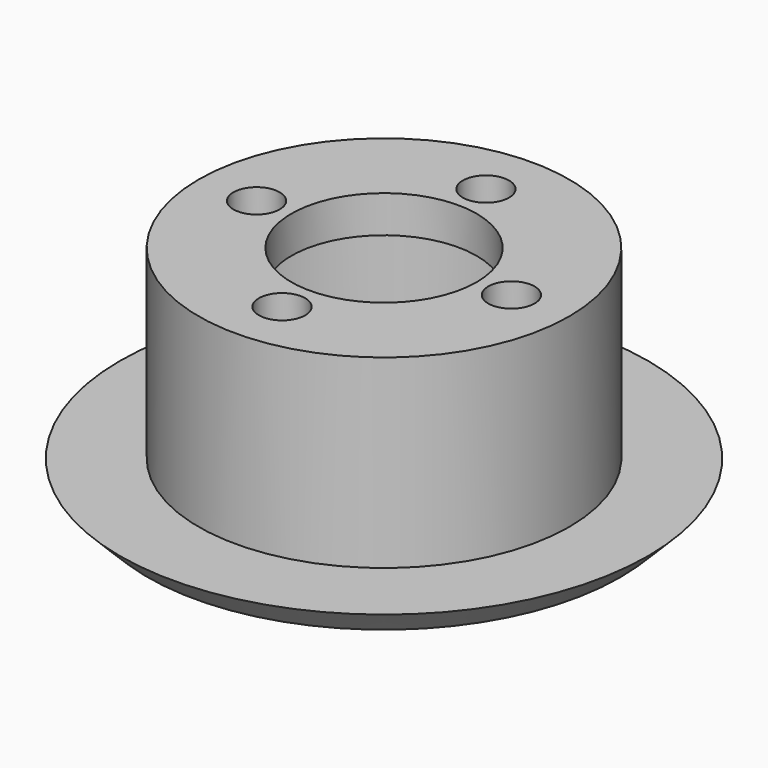
from build123d import *

# Parameters (mm, degrees)
F0_R     = 20
F0_R_2   = 17.5
F1_DEPTH = 23
F0_R_3   = 10
F2_DEPTH = 4
F3_R     = 28.5
F3_R_2   = 20
F4_DEPTH = 3
F5_R     = 2.5
F6_DEPTH = 4.001
F7_SIZE  = 2.99999
F8_SIZE  = 3


# Not quite as in the source:
# - a fillet or chamfer is up to 0.001 mm smaller than in the source, because OpenCascade refuses the exact size


with BuildPart() as f1:
    # F0 (on Top) → F1 (new body)
    with BuildSketch(Plane.XY):
        Circle(F0_R)
        Circle(F0_R_2, mode=Mode.SUBTRACT)
    extrude(amount=-F1_DEPTH)

    # F0 (on Top) → F2 (join)
    with BuildSketch(Plane.XY):
        Circle(F0_R_2)
        Circle(F0_R_3, mode=Mode.SUBTRACT)
    extrude(amount=-F2_DEPTH)

    # F3 (on face) → F4 (join)
    with BuildSketch(Plane(origin=(0, 0, -23), x_dir=(1, 0, 0), z_dir=(0, 0, -1))):
        Circle(F3_R)
        Circle(F3_R_2, mode=Mode.SUBTRACT)
    extrude(amount=-F4_DEPTH)

    # F5 (on face) → F6 (cut, through all)
    with BuildSketch(Plane(origin=(0, 0, -4), x_dir=(1, 0, 0), z_dir=(0, 0, -1))):
        with Locations((0, 13.75)):
            Circle(F5_R)
        with Locations((-13.75, 0)):
            Circle(F5_R)
        with Locations((0, -13.75)):
            Circle(F5_R)
        with Locations((13.75, 0)):
            Circle(F5_R)
    extrude(amount=-F6_DEPTH, mode=Mode.SUBTRACT)

    # F7 (size 3 in the source; OpenCascade refuses exactly that, so slightly less here)
    f7_edges = [f1.edges().sort_by_distance(p)[0] for p in [
        (-28.5, 0, -23),
    ]]
    chamfer(f7_edges, length=F7_SIZE)

    # F8
    f8_edges = [f1.edges().sort_by_distance(p)[0] for p in [
        (-17.5, 0, -23),
    ]]
    chamfer(f8_edges, length=F8_SIZE)


solid = f1.part
